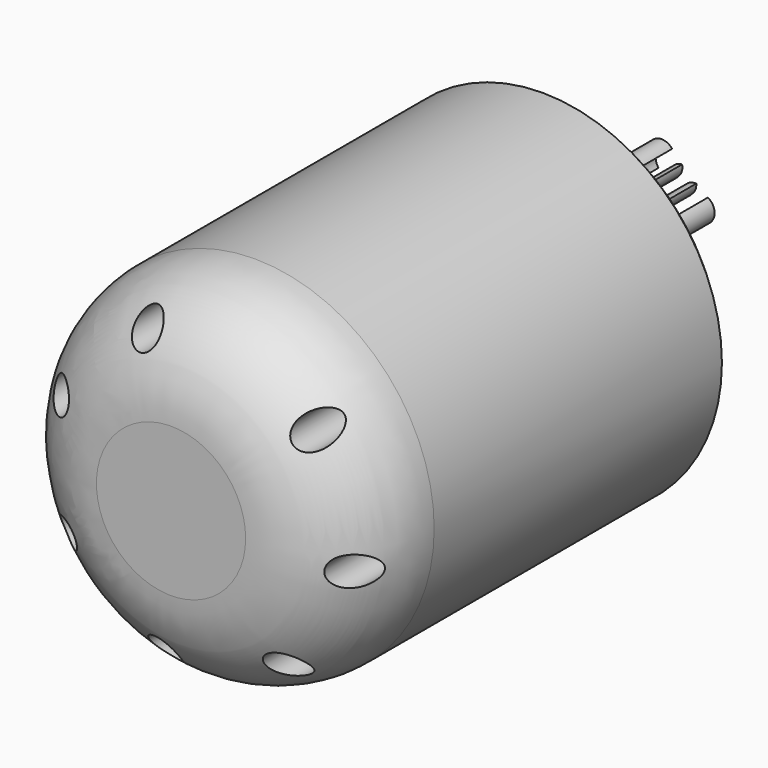
from build123d import *

# Parameters (mm, degrees)
F0_R     = 111.6181809064
F0_R_2   = 9.6407803701
F1_DEPTH = 296
F5_DEPTH = 25


# Not quite as in the source:
# - a fillet or chamfer that OpenCascade refuses, or shapes differently, is made with other operations: its cross-section is extruded or revolved along the edge and cut away or added


with BuildPart() as f1:
    # F0 (on Front) → F1 (new body)
    with BuildSketch(Plane.XZ):
        Circle(F0_R)
        with Locations((-16.8322412, -87.5481787514)):
            Circle(F0_R_2, mode=Mode.SUBTRACT)
        with Locations((-74.9043936204, -41.8695382418)):
            Circle(F0_R_2, mode=Mode.SUBTRACT)
        with Locations((55.8969753172, -74.5337963101)):
            Circle(F0_R_2, mode=Mode.SUBTRACT)
        with Locations((94.5249877968, -11.5513405195)):
            Circle(F0_R_2, mode=Mode.SUBTRACT)
        with Locations((-79.3874307759, 31.8787869147)):
            Circle(F0_R_2, mode=Mode.SUBTRACT)
        with Locations((-27.2758874883, 84.2553097252)):
            Circle(F0_R_2, mode=Mode.SUBTRACT)
        with Locations((73.1552572663, 59.1752294708)):
            Circle(F0_R_2, mode=Mode.SUBTRACT)
    extrude(amount=F1_DEPTH)

    # F2: fillet of radius 65.1837661841 on 1 edges, made by hand

    # F2_s1 → F2_t2 (revolve, cut)
    with BuildSketch(Plane.XY):
        with BuildLine():
            ThreePointArc((111.6181809064, -230.8162338159), (92.5262978144, -276.908116908), (46.4344147224, -296))
            Line((46.4344147224, -296), (111.6181809064, -296))
            Line((111.6181809064, -296), (111.6181809064, -230.8162338159))
        make_face()
    revolve(axis=Axis((0, -296, 0), (0, -1, 0)), mode=Mode.SUBTRACT)

    # F3: chamfer of 7 on 8 edges, made by hand

    # F3_s1 → F3_t2 (revolve, cut)
    with BuildSketch(Plane.XY.offset(84.2553097252)):
        Polygon((-17.6351071181, -7), (-10.6351071181, 0), (-17.6351071181, 0), align=None)
    revolve(axis=Axis((-27.2758874883, 0, 84.2553097252), (0, -1, 0)), mode=Mode.SUBTRACT)

    # F3_s3 → F3_t4 (revolve, cut)
    with BuildSketch(Plane.XY.offset(31.8787869147)):
        Polygon((-69.7466504057, -7), (-62.7466504057, 0), (-69.7466504057, 0), align=None)
    revolve(axis=Axis((-79.3874307759, 0, 31.8787869147), (0, -1, 0)), mode=Mode.SUBTRACT)

    # F3_s5 → F3_t6 (revolve, cut)
    with BuildSketch(Plane.XY):
        Polygon((111.6181809064, -7), (104.6181809064, 0), (111.6181809064, 0), align=None)
    revolve(axis=Axis((0, 0, 0), (0, -1, 0)), mode=Mode.SUBTRACT)

    # F3_s7 → F3_t8 (revolve, cut)
    with BuildSketch(Plane.XY.offset(-87.5481787514)):
        Polygon((-7.1914608299, -7), (-0.1914608299, 0), (-7.1914608299, 0), align=None)
    revolve(axis=Axis((-16.8322412, 0, -87.5481787514), (0, -1, 0)), mode=Mode.SUBTRACT)

    # F3_s9 → F3_t10 (revolve, cut)
    with BuildSketch(Plane.XY.offset(-41.8695382418)):
        Polygon((-65.2636132502, -7), (-58.2636132502, 0), (-65.2636132502, 0), align=None)
    revolve(axis=Axis((-74.9043936204, 0, -41.8695382418), (0, -1, 0)), mode=Mode.SUBTRACT)

    # F3_s11 → F3_t12 (revolve, cut)
    with BuildSketch(Plane.XY.offset(-74.5337963101)):
        Polygon((65.5377556874, -7), (72.5377556874, 0), (65.5377556874, 0), align=None)
    revolve(axis=Axis((55.8969753172, 0, -74.5337963101), (0, -1, 0)), mode=Mode.SUBTRACT)

    # F3_s13 → F3_t14 (revolve, cut)
    with BuildSketch(Plane.XY.offset(-11.5513405195)):
        Polygon((104.165768167, -7), (111.165768167, 0), (104.165768167, 0), align=None)
    revolve(axis=Axis((94.5249877968, 0, -11.5513405195), (0, -1, 0)), mode=Mode.SUBTRACT)

    # F3_s15 → F3_t16 (revolve, cut)
    with BuildSketch(Plane.XY.offset(59.1752294708)):
        Polygon((82.7960376364, -7), (89.7960376364, 0), (82.7960376364, 0), align=None)
    revolve(axis=Axis((73.1552572663, 0, 59.1752294708), (0, -1, 0)), mode=Mode.SUBTRACT)

    # F4 (on face) → F5, piece 3 (join)
    with BuildSketch(Plane(origin=(0, 0, 0), x_dir=(-1, 0, 0), z_dir=(0, 1, 0))):
        with BuildLine():
            ThreePointArc((-58.6073712589, 71.4413412829), (-56.284149618, 69.992802613), (-53.6162424185, 69.3780715775))
            ThreePointArc((-53.6162424185, 69.3780715775), (-53.4994770648, 70.1750058259), (-53.4604329494, 70.9795018801))
            ThreePointArc((-53.4604329494, 70.9795018801), (-53.6869817261, 72.906391019), (-54.3542722966, 74.7281894153))
            ThreePointArc((-54.3542722966, 74.7281894153), (-55.222843002, 75.7403261506), (-55.9182564321, 76.8784105071))
            ThreePointArc((-55.9182564321, 76.8784105071), (-58.3724078083, 78.5615548701), (-61.2622734735, 79.2718437982))
            ThreePointArc((-61.2622734735, 79.2718437982), (-61.3036475349, 76.2962561065), (-60.2937336183, 73.4969869509))
            ThreePointArc((-60.2937336183, 73.4969869509), (-59.3677818798, 72.5370654858), (-58.6073712589, 71.4413412829))
        make_face()
        with BuildLine():
            ThreePointArc((-44.8025613038, 77.6704134956), (-45.2568282643, 74.9608888065), (-46.5699506643, 72.5476768235))
            ThreePointArc((-46.5699506643, 72.5476768235), (-41.9817092657, 75.4817852348), (-40.1965741405, 80.6270980422))
            ThreePointArc((-40.1965741405, 80.6270980422), (-45.7948102708, 88.4805919011), (-55.0447064188, 85.7498347143))
            ThreePointArc((-55.0447064188, 85.7498347143), (-47.9650093158, 84.1930391898), (-44.8025613038, 77.6704134956))
        make_face()
    extrude(amount=F5_DEPTH)


with BuildPart() as f5:
    # F4 (on face) → F5 (new body)
    with BuildSketch(Plane(origin=(0, 0, 0), x_dir=(-1, 0, 0), z_dir=(0, 1, 0))):
        with BuildLine():
            ThreePointArc((-68.4185283557, 66.0003513789), (-67.3873974914, 65.154416995), (-66.5049226793, 64.154379972))
            ThreePointArc((-66.5049226793, 64.154379972), (-64.0292447566, 62.9853453728), (-61.3080110738, 62.6844960501))
            ThreePointArc((-61.3080110738, 62.6844960501), (-61.2892519266, 63.0063624098), (-61.2829957366, 63.3287142659))
            ThreePointArc((-61.2829957366, 63.3287142659), (-61.6352552844, 65.722224105), (-62.6621614287, 67.9127582658))
            ThreePointArc((-62.6621614287, 67.9127582658), (-63.6423610727, 68.8172163903), (-64.4651958955, 69.8668728558))
            ThreePointArc((-64.4651958955, 69.8668728558), (-67.0981543121, 71.2537268139), (-70.050939251, 71.6237200959))
            ThreePointArc((-70.050939251, 71.6237200959), (-69.7465889094, 68.6634490282), (-68.4185283557, 66.0003513789))
        make_face()
    extrude(amount=F5_DEPTH)


with BuildPart() as f5b:
    # F4 (on face) → F5, piece 2 (new body)
    with BuildSketch(Plane(origin=(0, 0, 0), x_dir=(-1, 0, 0), z_dir=(0, 1, 0))):
        with BuildLine():
            ThreePointArc((-77.3255812582, 66.3604425946), (-78.5656998997, 52.8707865657), (-65.4204325641, 56.1435011421))
            ThreePointArc((-65.4204325641, 56.1435011421), (-75.0011991894, 57.0242713608), (-77.3255812582, 66.3604425946))
        make_face()
    extrude(amount=F5_DEPTH)


solid = Compound([f1.part, f5.part, f5b.part])
